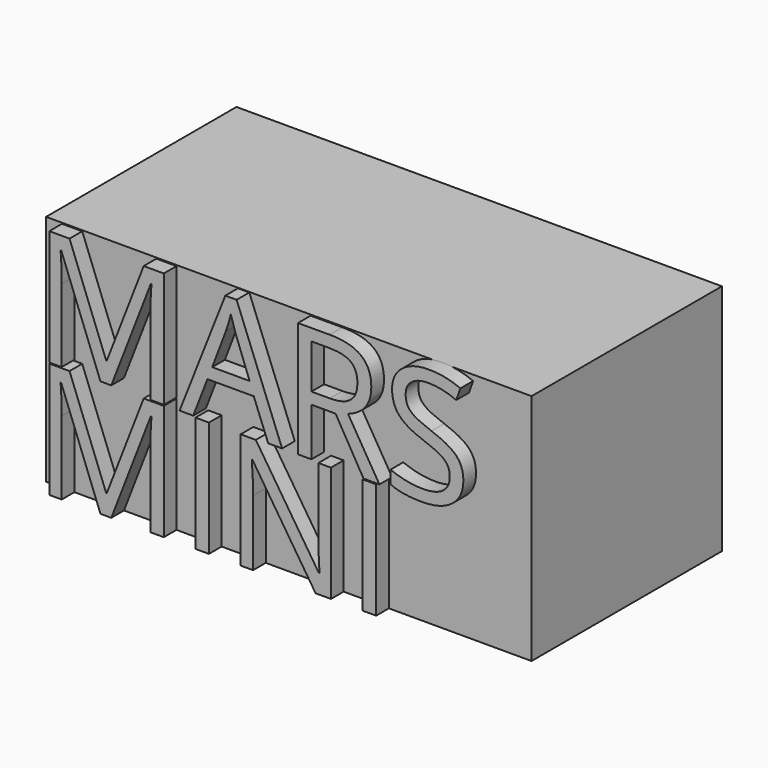
from build123d import *

# Parameters (mm, degrees)
F2_W         = 306
F2_H         = 147
F0_DEPTH     = 150
F1_TEXT_SIZE = 102.0833333333
F3_DEPTH     = 10


# Not quite as in the source:
# - Text() gives the source's letters only with a copy of the font that has no kerning and outlines rounded to 1/6400 em; it was checked with that copy


with BuildPart() as f0:
    # F2 (on Front) → F0 (new body)
    with BuildSketch(Plane.XZ):
        with Locations((153, 73.5)):
            Rectangle(F2_W, F2_H)
    extrude(amount=F0_DEPTH)

    # F1 (on face) → F3 (join)
    with BuildSketch(Plane.XZ.offset(150)):
        with Locations((0, 73.5)):
            Text('MARS', F1_TEXT_SIZE, font='Open Sans', text_align=(TextAlign.LEFT, TextAlign.BOTTOM))
        with Locations((0, 0)):
            Text('MINI', F1_TEXT_SIZE, font='Open Sans', text_align=(TextAlign.LEFT, TextAlign.BOTTOM))
    extrude(amount=F3_DEPTH)


solid = f0.part
